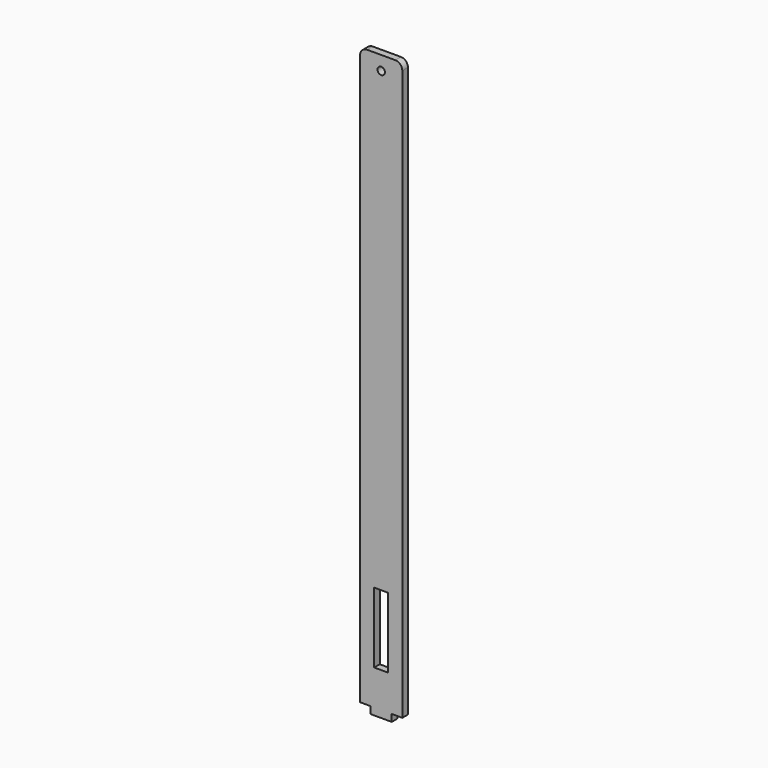
from build123d import *

# Parameters (mm, degrees)
F0_W     = 15
F0_H     = 5
F1_DEPTH = 2.5
F3_D     = 5.25
F4_R     = 5
F5_W     = 10
F5_H     = 50
F6_DEPTH = 10


with BuildPart() as f1:
    # F0 (on Front) → F1 (new body, symmetric)
    with BuildSketch(Plane.XZ):
        Polygon((15, -205), (15, 205), (-15, 205), (-15, -205), (-7.5, -205), (-7.5, -200), (7.5, -200), (7.5, -205), align=None)
        with Locations((0, -207.5)):
            Rectangle(F0_W, F0_H)
        with Locations((0, -202.5)):
            Rectangle(F0_W, F0_H)
    extrude(amount=F1_DEPTH, both=True)

    # F3 (through all)
    with Locations(Plane.XZ.offset(2.5)):
        with Locations((0, 195)):
            Hole(F3_D / 2)

    # F4
    f4_edges = [f1.edges().sort_by_distance(p)[0] for p in [
        (15, 0, 205),
        (-15, 0, 205),
    ]]
    fillet(f4_edges, radius=F4_R)

    # F5 (on face) → F6 (cut)
    with BuildSketch(Plane.XZ.offset(2.5)):
        with Locations((0, -155)):
            Rectangle(F5_W, F5_H)
    extrude(amount=-F6_DEPTH, mode=Mode.SUBTRACT)


solid = f1.part
